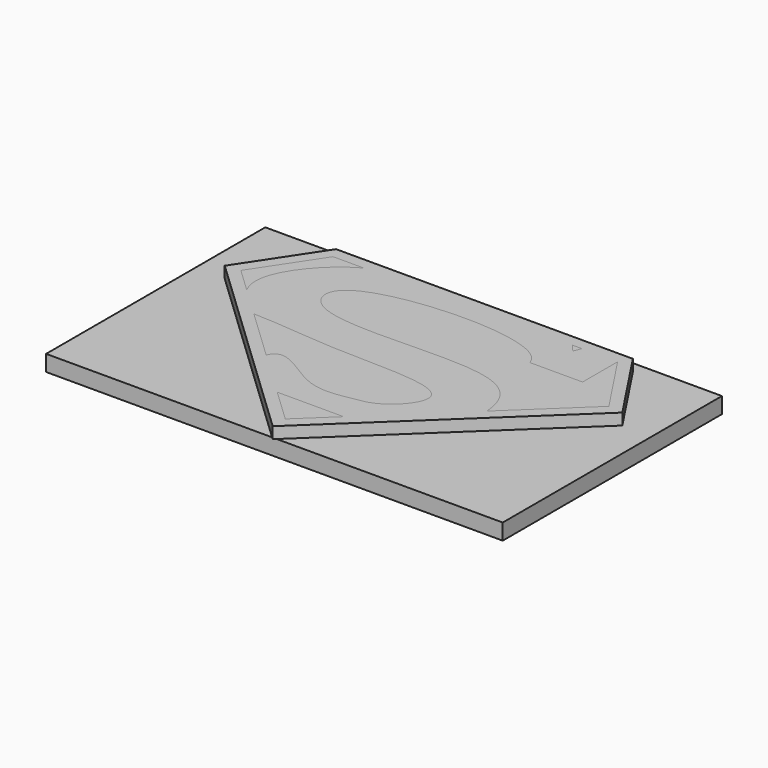
from build123d import *

# Parameters (mm, degrees)
F0_W     = 254
F0_H     = 152.4
F1_DEPTH = 8.89
F3_DEPTH = 6.35
F4_DEPTH = 6.35


with BuildPart() as f1:
    # F0 (on Top) → F1 (new body)
    with BuildSketch(Plane.XY):
        Rectangle(F0_W, F0_H)
    extrude(amount=-F1_DEPTH)


with BuildPart() as f3:
    # F2 (on face) → F3 (new body)
    with BuildSketch(Plane.XY):
        Polygon((-110.5765039644, 27.4807295846), (0, -77.3934653874), (110.5765039644, 27.4807295846), (82.55, 69.85), (0, 69.85), (-82.55, 69.85), align=None)
        Polygon((0, -68.6416965639), (-18.4294173274, -51.1626640686), (18.4294173274, -51.1626640686), align=None, mode=Mode.SUBTRACT)
        with BuildLine():
            Line((-44.0000207675, -26.9107085936), (-72.3739413137, 0))
            add(Edge.make_bspline(
                [(-72.3739413137, 0), (-56.4772636932, -0.1623677252), (-25.4767474165, -5.51335001), (53.4650384253, -1.948212177), (28.0139967905, -31.6587429979), (16.7418438941, -34.3451872468)],
                knots=[0, 0, 0, 0, 0.3610325629, 0.7321442872, 1, 1, 1, 1], degree=3))
            add(Edge.make_bspline(
                [(16.7418438941, -34.3451872468), (6.3339606859, -35.8872525394), (-12.5582004687, -43.0800227139), (-39.5378135145, -15.8403627574), (-44.0000207675, -26.9107085936)],
                knots=[0, 0, 0, 0, 0.5062543881, 1, 1, 1, 1], degree=3))
        make_face(mode=Mode.SUBTRACT)
        with BuildLine():
            Line((-102.34071652, 28.4214214864), (-79.1368730236, 63.5))
            Line((-79.1368730236, 63.5), (-61.8954822743, 63.5))
            add(Edge.make_bspline(
                [(-61.8954822743, 63.5), (-72.6268264588, 58.5622080867), (-95.101295313, 37.3717973696), (-90.5552589798, 19.7811521388)],
                knots=[0, 0, 0, 0, 50.9395259322, 50.9395259322, 50.9395259322, 50.9395259322], degree=3))
            Line((-90.5552589798, 19.7811521388), (-88.9901484483, 15.7593275628))
            Line((-88.9901484483, 15.7593275628), (-102.34071652, 28.4214214864))
        make_face(mode=Mode.SUBTRACT)
        with BuildLine():
            Line((102.34071652, 28.4214214864), (63.7637178758, -8.1662036618))
            add(Edge.make_bspline(
                [(49.7100912035, 39.1332991421), (44.9893101786, 59.2620450287), (-65.5701214452, 56.8028238808), (-58.1526178236, 11.8855718778), (32.4692170914, 25.4260499791), (62.1978511511, 11.5267576353), (63.7637178758, -8.1662036618)],
                knots=[0, 0, 0, 0, 0.3358949045, 0.4796056591, 0.7830399215, 1, 1, 1, 1], degree=3))
            Line((49.7100912035, 39.1332991421), (79.1368730236, 39.1332991421))
            Line((79.1368730236, 39.1332991421), (79.1368730236, 63.5))
            Line((79.1368730236, 63.5), (102.34071652, 28.4214214864))
        make_face(mode=Mode.SUBTRACT)
        Polygon((54.0717579424, 63.5), (59.3367516994, 63.5), (57.6373636723, 59.224486351), align=None, mode=Mode.SUBTRACT)
    extrude(amount=F3_DEPTH)


with BuildPart() as f4:
    # F2 (on face) → F4 (new body, through all)
    with BuildSketch(Plane.XY):
        Polygon((57.6373636723, 59.224486351), (59.3367516994, 63.5), (54.0717579424, 63.5), align=None)
    extrude(amount=F4_DEPTH)


with BuildPart() as f4b:
    # F2 (on face) → F4, piece 2 (new body, through all)
    with BuildSketch(Plane.XY):
        with BuildLine():
            add(Edge.make_bspline(
                [(49.7100912035, 39.1332991421), (44.9893101786, 59.2620450287), (-65.5701214452, 56.8028238808), (-58.1526178236, 11.8855718778), (32.4692170914, 25.4260499791), (62.1978511511, 11.5267576353), (63.7637178758, -8.1662036618)],
                knots=[0, 0, 0, 0, 0.3358949045, 0.4796056591, 0.7830399215, 1, 1, 1, 1], degree=3))
            Line((63.7637178758, -8.1662036618), (102.34071652, 28.4214214864))
            Line((102.34071652, 28.4214214864), (79.1368730236, 63.5))
            Line((79.1368730236, 63.5), (79.1368730236, 39.1332991421))
            Line((79.1368730236, 39.1332991421), (49.7100912035, 39.1332991421))
        make_face()
    extrude(amount=F4_DEPTH)


with BuildPart() as f4c:
    # F2 (on face) → F4, piece 3 (new body, through all)
    with BuildSketch(Plane.XY):
        Polygon((18.4294173274, -51.1626640686), (-18.4294173274, -51.1626640686), (0, -68.6416965639), align=None)
    extrude(amount=F4_DEPTH)


with BuildPart() as f4d:
    # F2 (on face) → F4, piece 4 (new body, through all)
    with BuildSketch(Plane.XY):
        with BuildLine():
            add(Edge.make_bspline(
                [(-72.3739413137, 0), (-56.4772636932, -0.1623677252), (-25.4767474165, -5.51335001), (53.4650384253, -1.948212177), (28.0139967905, -31.6587429979), (16.7418438941, -34.3451872468)],
                knots=[0, 0, 0, 0, 0.3610325629, 0.7321442872, 1, 1, 1, 1], degree=3))
            Line((-72.3739413137, 0), (-44.0000207675, -26.9107085936))
            add(Edge.make_bspline(
                [(16.7418438941, -34.3451872468), (6.3339606859, -35.8872525394), (-12.5582004687, -43.0800227139), (-39.5378135145, -15.8403627574), (-44.0000207675, -26.9107085936)],
                knots=[0, 0, 0, 0, 0.5062543881, 1, 1, 1, 1], degree=3))
        make_face()
    extrude(amount=F4_DEPTH)


with BuildPart() as f4e:
    # F2 (on face) → F4, piece 5 (new body, through all)
    with BuildSketch(Plane.XY):
        with BuildLine():
            Line((-61.8954822743, 63.5), (-79.1368730236, 63.5))
            Line((-79.1368730236, 63.5), (-102.34071652, 28.4214214864))
            Line((-102.34071652, 28.4214214864), (-88.9901484483, 15.7593275628))
            add(Edge.make_bspline(
                [(-90.5552589798, 19.7811521388), (-90.2023942784, 18.4157609891), (-89.6867334414, 17.0720581056), (-88.9901484483, 15.7593275628)],
                knots=[50.9395259322, 50.9395259322, 50.9395259322, 50.9395259322, 54.8934671872, 54.8934671872, 54.8934671872, 54.8934671872], degree=3))
            add(Edge.make_bspline(
                [(-61.8954822743, 63.5), (-72.6268264588, 58.5622080867), (-95.101295313, 37.3717973696), (-90.5552589798, 19.7811521388)],
                knots=[0, 0, 0, 0, 50.9395259322, 50.9395259322, 50.9395259322, 50.9395259322], degree=3))
        make_face()
        with BuildLine():
            Line((-88.9901484483, 15.7593275628), (-90.5552589798, 19.7811521388))
            add(Edge.make_bspline(
                [(-90.5552589798, 19.7811521388), (-90.2023942784, 18.4157609891), (-89.6867334414, 17.0720581056), (-88.9901484483, 15.7593275628)],
                knots=[50.9395259322, 50.9395259322, 50.9395259322, 50.9395259322, 54.8934671872, 54.8934671872, 54.8934671872, 54.8934671872], degree=3))
        make_face()
    extrude(amount=F4_DEPTH)


solid = Compound([f1.part, f3.part, f4.part, f4b.part, f4c.part, f4d.part, f4e.part])
